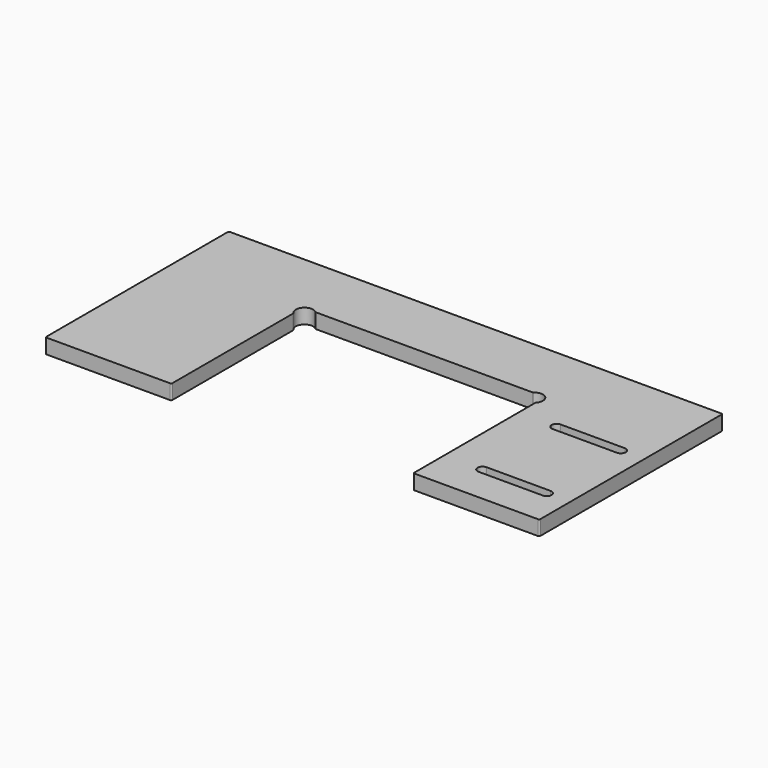
from build123d import *

# Parameters (mm, degrees)
F0_W     = 60
F0_H     = 8
F1_DEPTH = 12
F2_R     = 1
F3_R     = 3.99999


# Not quite as in the source:
# - a fillet or chamfer is up to 0.001 mm smaller than in the source, because OpenCascade refuses the exact size


with BuildPart() as f1:
    # F0 (on Top) → F1 (new body)
    with BuildSketch(Plane.XY):
        with BuildLine():
            Line((200, 0), (-200, 0))
            Line((-200, 0), (-200, -185.5))
            Line((-200, -185.5), (-98, -185.5))
            Line((-98, -185.5), (-98, -61.8994949366))
            ThreePointArc((-98, -61.8994949366), (-98, -52), (-88.1005050634, -52))
            Line((-88.1005050634, -52), (88.1005050634, -52))
            ThreePointArc((88.1005050634, -52), (98, -52), (98, -61.8994949366))
            Line((98, -61.8994949366), (98, -185.5))
            Line((98, -185.5), (200, -185.5))
            Line((200, -185.5), (200, 0))
        make_face()
        with Locations((155, -154.25)):
            Rectangle(F0_W, F0_H, mode=Mode.SUBTRACT)
        with Locations((155, -79.25)):
            Rectangle(F0_W, F0_H, mode=Mode.SUBTRACT)
    extrude(amount=F1_DEPTH)

    # F2
    f2_edges = [f1.edges().sort_by_distance(p)[0] for p in [
        (-98, -185.5, 6),
        (-98, -61.899495, 6),
        (-88.100505, -52, 6),
        (88.100505, -52, 6),
        (98, -61.899495, 6),
        (98, -185.5, 6),
        (200, -185.5, 6),
        (200, 0, 6),
        (-200, 0, 6),
        (-200, -185.5, 6),
    ]]
    fillet(f2_edges, radius=F2_R)

    # F3 (radius 4 in the source; OpenCascade refuses exactly that, so slightly less here)
    f3_edges = [f1.edges().sort_by_distance(p)[0] for p in [
        (125, -158.25, 6),
        (125, -150.25, 6),
        (185, -158.25, 6),
        (185, -150.25, 6),
        (125, -83.25, 6),
        (125, -75.25, 6),
        (185, -83.25, 6),
        (185, -75.25, 6),
    ]]
    fillet(f3_edges, radius=F3_R)


solid = f1.part
